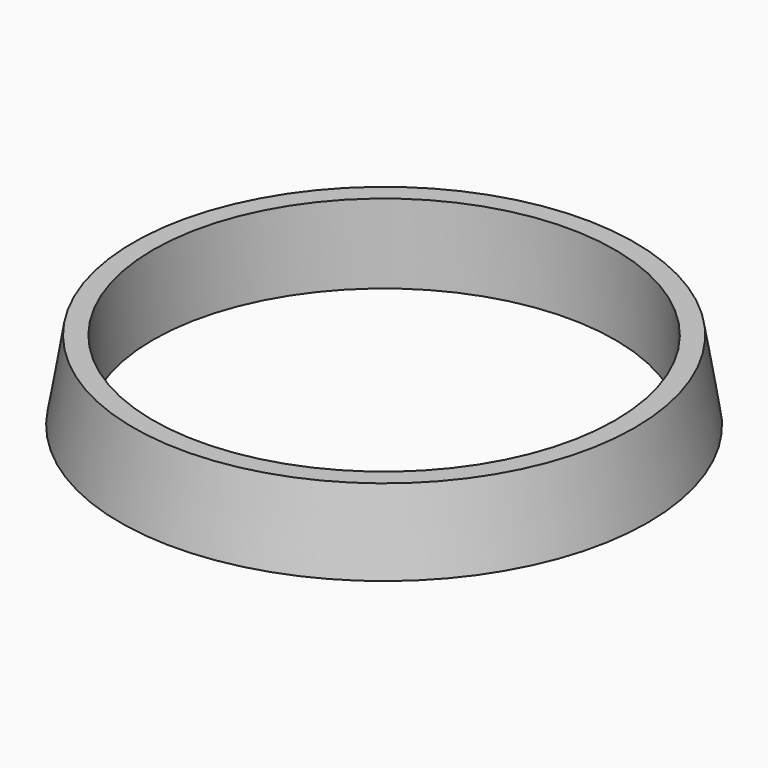
from build123d import *

# Parameters (mm, degrees)
F0_R     = 2
F1_DEPTH = 0.6
F2_D     = 3.5
F3_SIZE2 = 0.59999
F3_SIZE  = 0.09999


# Not quite as in the source:
# - a fillet or chamfer is up to 0.001 mm smaller than in the source, because OpenCascade refuses the exact size


with BuildPart() as f1:
    # F0 (on Top) → F1 (new body)
    with BuildSketch(Plane.XY):
        Circle(F0_R)
    extrude(amount=F1_DEPTH)

    # F2 (through all)
    with Locations(Plane(origin=(0, 0, 0), x_dir=(1, 0, 0), z_dir=(0, 0, -1))):
        with Locations((0, 0)):
            Hole(F2_D / 2)

    # F3 (size 0.1 and 0.6 in the source; OpenCascade refuses exactly that, so slightly less here)
    f3_edges = [f1.edges().sort_by_distance(p)[0] for p in [
        (-2, 0, 0.6),
    ]]
    f3_side = f1.faces().sort_by_distance((-1.943431, 0, 0.6))[0]
    chamfer(f3_edges, length=F3_SIZE, length2=F3_SIZE2, reference=f3_side)


solid = f1.part
